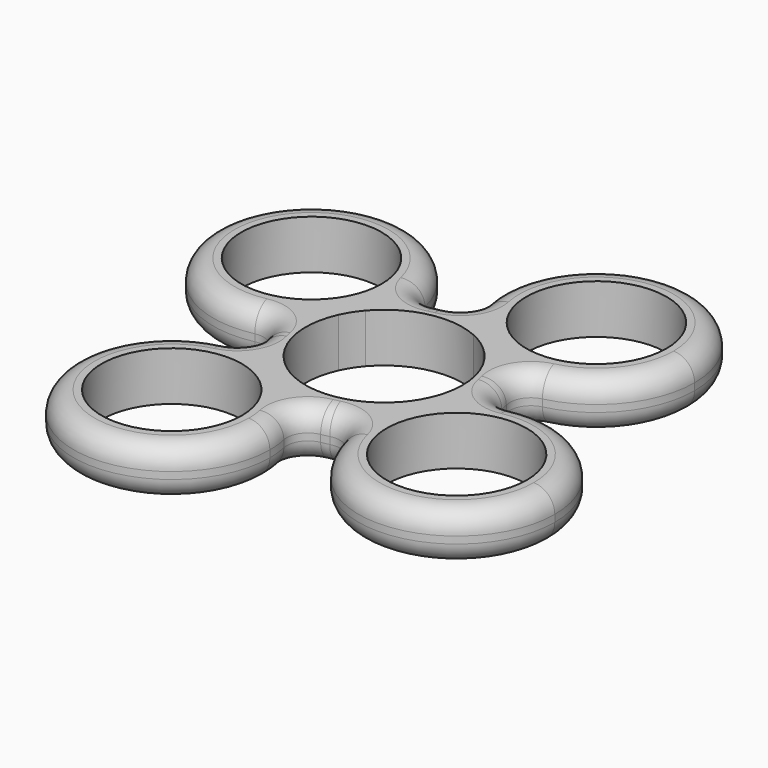
from build123d import *

# Parameters (mm, degrees)
F0_R     = 10
F1_DEPTH = 7
F2_R     = 3


with BuildPart() as f1:
    # F0 (on Top) → F1 (new body)
    with BuildSketch(Plane.XY):
        with BuildLine():
            ThreePointArc((-8.5099476782, 7.2815376477), (-2.4295810376, 10.9333039829), (4.6251408746, 10.2003956732))
            ThreePointArc((4.6251408746, 10.2003956732), (2.4988162565, 12.3345005205), (0.87828133, 14.8740923053))
            ThreePointArc((0.87828133, 14.8740923053), (-3.2322104876, 14.5451990486), (-7.0951390366, 13.1022517932))
            ThreePointArc((-7.0951390366, 13.1022517932), (-7.4875831187, 10.1153390855), (-8.5099476782, 7.2815376477))
        make_face()
        with BuildLine():
            ThreePointArc((4.6251408746, 10.2003956732), (6.0130401599, 9.4489866142), (7.2815376477, 8.5099476782))
            ThreePointArc((7.2815376477, 8.5099476782), (10.1153390855, 7.4875831187), (13.1022517932, 7.0951390366))
            ThreePointArc((13.1022517932, 7.0951390366), (7.999490927, 12.570526835), (0.87828133, 14.8740923053))
            ThreePointArc((0.87828133, 14.8740923053), (2.4988162565, 12.3345005205), (4.6251408746, 10.2003956732))
        make_face()
        with BuildLine():
            ThreePointArc((7.2815376477, 8.5099476782), (10.1733284046, 4.6843771382), (11.2, 0))
            ThreePointArc((11.2, 0), (10.9472469493, -2.3659637001), (10.2003956732, -4.6251408746))
            ThreePointArc((10.2003956732, -4.6251408746), (12.3345005205, -2.4988162565), (14.8740923053, -0.87828133))
            ThreePointArc((14.8740923053, -0.87828133), (14.893521668, -0.4393316809), (14.9, 0))
            ThreePointArc((14.9, 0), (14.4435721295, 3.6596754147), (13.1022517932, 7.0951390366))
            ThreePointArc((13.1022517932, 7.0951390366), (10.1153390855, 7.4875831187), (7.2815376477, 8.5099476782))
        make_face()
        with BuildLine():
            ThreePointArc((-10.2003956732, 4.6251408746), (-9.4489866142, 6.0130401599), (-8.5099476782, 7.2815376477))
            ThreePointArc((-8.5099476782, 7.2815376477), (-7.4875831187, 10.1153390855), (-7.0951390366, 13.1022517932))
            ThreePointArc((-7.0951390366, 13.1022517932), (-12.570526835, 7.999490927), (-14.8740923053, 0.87828133))
            ThreePointArc((-14.8740923053, 0.87828133), (-12.3345005205, 2.4988162565), (-10.2003956732, 4.6251408746))
        make_face()
        with BuildLine():
            ThreePointArc((-14.8740923053, 0.87828133), (-12.570526835, 7.999490927), (-7.0951390366, 13.1022517932))
            ThreePointArc((-7.0951390366, 13.1022517932), (-7.0924007725, 13.2620977947), (-7.0914879781, 13.4219646426))
            ThreePointArc((-7.0914879781, 13.4219646426), (-32.9877802455, 20.8029015947), (-14.8740923053, 0.87828133))
        make_face()
        with Locations((-21.0914879781, 13.4219646426)):
            Circle(F0_R, mode=Mode.SUBTRACT)
        with BuildLine():
            ThreePointArc((-7.2815376477, -8.5099476782), (-10.9333039829, -2.4295810376), (-10.2003956732, 4.6251408746))
            ThreePointArc((-10.2003956732, 4.6251408746), (-12.3345005205, 2.4988162565), (-14.8740923053, 0.87828133))
            ThreePointArc((-14.8740923053, 0.87828133), (-14.5451990486, -3.2322104876), (-13.1022517932, -7.0951390366))
            ThreePointArc((-13.1022517932, -7.0951390366), (-10.1153390855, -7.4875831187), (-7.2815376477, -8.5099476782))
        make_face()
        with BuildLine():
            ThreePointArc((0.5780353574, -21.0914879781), (0.2090948609, -17.8986496152), (-0.87828133, -14.8740923053))
            ThreePointArc((-0.87828133, -14.8740923053), (-7.999490927, -12.570526835), (-13.1022517932, -7.0951390366))
            ThreePointArc((-13.1022517932, -7.0951390366), (-23.4338570685, -30.8772945394), (0.5780353574, -21.0914879781))
        make_face()
        with Locations((-13.4219646426, -21.0914879781)):
            Circle(F0_R, mode=Mode.SUBTRACT)
        with BuildLine():
            ThreePointArc((-0.87828133, -14.8740923053), (-2.4988162565, -12.3345005205), (-4.6251408746, -10.2003956732))
            ThreePointArc((-4.6251408746, -10.2003956732), (-6.0130401599, -9.4489866142), (-7.2815376477, -8.5099476782))
            ThreePointArc((-7.2815376477, -8.5099476782), (-10.1153390855, -7.4875831187), (-13.1022517932, -7.0951390366))
            ThreePointArc((-13.1022517932, -7.0951390366), (-7.999490927, -12.570526835), (-0.87828133, -14.8740923053))
        make_face()
        with BuildLine():
            ThreePointArc((7.0951390366, -13.1022517932), (7.4875831187, -10.1153390855), (8.5099476782, -7.2815376477))
            ThreePointArc((8.5099476782, -7.2815376477), (2.4295810376, -10.9333039829), (-4.6251408746, -10.2003956732))
            ThreePointArc((-4.6251408746, -10.2003956732), (-2.4988162565, -12.3345005205), (-0.87828133, -14.8740923053))
            ThreePointArc((-0.87828133, -14.8740923053), (3.2322104876, -14.5451990486), (7.0951390366, -13.1022517932))
        make_face()
        with BuildLine():
            ThreePointArc((14.8740923053, -0.87828133), (12.3345005205, -2.4988162565), (10.2003956732, -4.6251408746))
            ThreePointArc((10.2003956732, -4.6251408746), (9.4489866142, -6.0130401599), (8.5099476782, -7.2815376477))
            ThreePointArc((8.5099476782, -7.2815376477), (7.4875831187, -10.1153390855), (7.0951390366, -13.1022517932))
            ThreePointArc((7.0951390366, -13.1022517932), (12.570526835, -7.999490927), (14.8740923053, -0.87828133))
        make_face()
        with BuildLine():
            ThreePointArc((35.0914879781, -13.4219646426), (28.4724249302, -1.5256723753), (14.8740923053, -0.87828133))
            ThreePointArc((14.8740923053, -0.87828133), (12.570526835, -7.999490927), (7.0951390366, -13.1022517932))
            ThreePointArc((7.0951390366, -13.1022517932), (20.9316211301, -27.4210518483), (35.0914879781, -13.4219646426))
        make_face()
        with Locations((21.0914879781, -13.4219646426)):
            Circle(F0_R, mode=Mode.SUBTRACT)
        with BuildLine():
            ThreePointArc((0.87828133, 14.8740923053), (7.999490927, 12.570526835), (13.1022517932, 7.0951390366))
            ThreePointArc((13.1022517932, 7.0951390366), (23.2077712039, 11.0795955523), (27.4219646426, 21.0914879781))
            ThreePointArc((27.4219646426, 21.0914879781), (10.2291262797, 34.7225474816), (0.87828133, 14.8740923053))
        make_face()
        with Locations((13.4219646426, 21.0914879781)):
            Circle(F0_R, mode=Mode.SUBTRACT)
    extrude(amount=F1_DEPTH)

    # F2
    f2_edges = [f1.edges().sort_by_distance(p)[0] for p in [
        (-20.938265, -32.902721, 0),
        (32.902721, -20.938265, 0),
        (20.938265, 32.902721, 0),
        (-32.902721, 20.938265, 0),
        (20.938265, 32.902721, 7),
        (-32.902721, 20.938265, 7),
        (-20.938265, -32.902721, 7),
        (32.902721, -20.938265, 7),
        (-14.874092, 0.878281, 3.5),
        (-13.102252, -7.095139, 3.5),
        (-14.545199, -3.23221, 0),
        (-14.545199, -3.23221, 7),
        (0.878281, 14.874092, 3.5),
        (-7.095139, 13.102252, 3.5),
        (-3.23221, 14.545199, 0),
        (-3.23221, 14.545199, 7),
        (-0.878281, -14.874092, 3.5),
        (7.095139, -13.102252, 3.5),
        (3.23221, -14.545199, 0),
        (3.23221, -14.545199, 7),
        (14.874092, -0.878281, 3.5),
        (13.102252, 7.095139, 3.5),
        (14.545199, 3.23221, 0),
        (14.545199, 3.23221, 7),
    ]]
    fillet(f2_edges, radius=F2_R)


solid = f1.part
